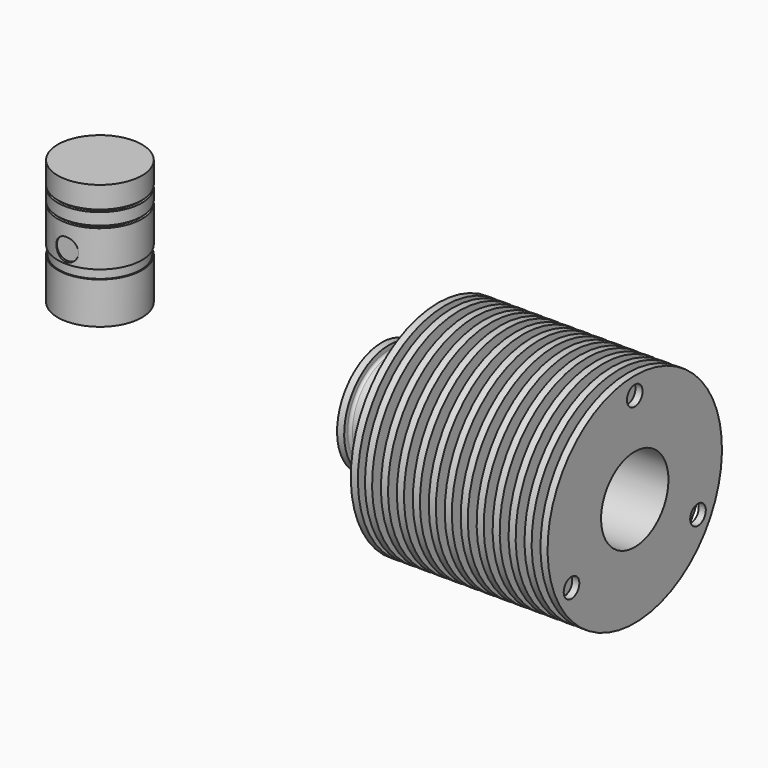
from build123d import *

# Parameters (mm, degrees)
F2_R      = 1.25
F3_DEPTH  = 5
F4_R      = 4.35
F5_DEPTH  = 4
F6_DEPTH  = 9.4
F7_R      = 1.25
F8_DEPTH  = 4.5
F12_D     = 2.2
F13_R     = 0.5
F14_DEPTH = 6.5
F16_R     = 0.5
F17_DEPTH = 6.5
F19_R     = 0.5
F20_DEPTH = 6.5


# Not quite as in the source:
# - a feature names something its author has since deleted; it is built from what else it names


with BuildPart() as f1:
    # F0 (on Front) → F1 (revolve)
    with BuildSketch(Plane.XZ):
        Polygon((-4.7528314651, -0.0212201326), (-0.0028314651, -0.0212201326), (-0.0028314651, 14.0787798674), (-4.7528314651, 14.0787798674), (-4.7528314651, 11.6291058475), (-4.6228314651, 11.4991058475), (-4.7528314651, 11.3691058475), (-4.7528314651, 10.0291058475), (-4.6228314651, 9.8991058475), (-4.7528314651, 9.7691058475), (-4.7528314651, 5.6787798674), (-4.6228314651, 5.6787798674), (-4.6228314651, 4.6787798674), (-4.7528314651, 4.6787798674), align=None)
    revolve(axis=Axis((-0.0028314651, 0, 3.8338128439), (0, 0, -1)))

    # F2 (on Front) → F3 (cut, symmetric)
    with BuildSketch(Plane.XZ):
        with Locations((0, 7.1287798674)):
            Circle(F2_R)
    extrude(amount=F3_DEPTH, both=True, mode=Mode.SUBTRACT)

    # F4 (on face) → F5 (cut)
    with BuildSketch(Plane(origin=(0, 0, -0.0212201326), x_dir=(1, 0, 0), z_dir=(0, 0, -1))):
        Circle(F4_R)
        with BuildLine():
            ThreePointArc((-2.8, 1), (-2.5071067812, 1.7071067812), (-1.8, 2))
            Line((-1.8, 2), (1.8, 2))
            ThreePointArc((1.8, 2), (2.5071067812, 1.7071067812), (2.8, 1))
            Line((2.8, 1), (2.8, -1))
            ThreePointArc((2.8, -1), (2.5071067812, -1.7071067812), (1.8, -2))
            Line((1.8, -2), (-1.8, -2))
            ThreePointArc((-1.8, -2), (-2.5071067812, -1.7071067812), (-2.8, -1))
            Line((-2.8, -1), (-2.8, 1))
        make_face(mode=Mode.SUBTRACT)
    extrude(amount=-F5_DEPTH, mode=Mode.SUBTRACT)

    # F6 (cut): a face of the model
    f6_faces = [f1.faces().sort_by_distance(p)[0] for p in [
        (0, 0, -0.0212201326),
    ]]
    extrude(f6_faces, amount=-F6_DEPTH, mode=Mode.SUBTRACT)


with BuildPart() as f8:
    # F7 (on Front) → F8 (new body, symmetric)
    with BuildSketch(Plane.XZ):
        with Locations((0, 7.1287798674)):
            Circle(F7_R)
    extrude(amount=F8_DEPTH, both=True)


with BuildPart() as f10:
    # F9 (on Front) → F10 (revolve)
    with BuildSketch(Plane.XZ):
        with BuildLine():
            Line((31.7983374715, 6.3), (31.7983374715, 4.75))
            Line((31.7983374715, 4.75), (60.3483374715, 4.75))
            Line((60.3483374715, 4.75), (60.3483374715, 12.3))
            Line((60.3483374715, 12.3), (59.5483374715, 12.3))
            Line((59.5483374715, 12.3), (59.5483374715, 6.75))
            Line((59.5483374715, 6.75), (58.5483374715, 6.75))
            Line((58.5483374715, 6.75), (58.5483374715, 12.3))
            Line((58.5483374715, 12.3), (57.7483374715, 12.3))
            Line((57.7483374715, 12.3), (57.7483374715, 6))
            Line((57.7483374715, 6), (56.7483374715, 6))
            Line((56.7483374715, 6), (56.7483374715, 12.3))
            Line((56.7483374715, 12.3), (55.9483374715, 12.3))
            Line((55.9483374715, 12.3), (55.9483374715, 6))
            Line((55.9483374715, 6), (54.9483374715, 6))
            Line((54.9483374715, 6), (54.9483374715, 12.3))
            Line((54.9483374715, 12.3), (54.1483374715, 12.3))
            Line((54.1483374715, 12.3), (54.1483374715, 6))
            Line((54.1483374715, 6), (53.1483374715, 6))
            Line((53.1483374715, 6), (53.1483374715, 12.3))
            Line((53.1483374715, 12.3), (52.3483374715, 12.3))
            Line((52.3483374715, 12.3), (52.3483374715, 6))
            Line((52.3483374715, 6), (51.3483374715, 6))
            Line((51.3483374715, 6), (51.3483374715, 12.3))
            Line((51.3483374715, 12.3), (50.5483374715, 12.3))
            Line((50.5483374715, 12.3), (50.5483374715, 6))
            Line((50.5483374715, 6), (49.5483374715, 6))
            Line((49.5483374715, 6), (49.5483374715, 12.3))
            Line((49.5483374715, 12.3), (48.7483374715, 12.3))
            Line((48.7483374715, 12.3), (48.7483374715, 6))
            Line((48.7483374715, 6), (47.7483374715, 6))
            Line((47.7483374715, 6), (47.7483374715, 12.3))
            Line((47.7483374715, 12.3), (46.9483374715, 12.3))
            Line((46.9483374715, 12.3), (46.9483374715, 6))
            Line((46.9483374715, 6), (45.9483374715, 6))
            Line((45.9483374715, 6), (45.9483374715, 12.3))
            Line((45.9483374715, 12.3), (45.1483374715, 12.3))
            Line((45.1483374715, 12.3), (45.1483374715, 6))
            Line((45.1483374715, 6), (44.1483374715, 6))
            Line((44.1483374715, 6), (44.1483374715, 12.3))
            Line((44.1483374715, 12.3), (43.3483374715, 12.3))
            Line((43.3483374715, 12.3), (43.3483374715, 6))
            Line((43.3483374715, 6), (42.3483374715, 6))
            Line((42.3483374715, 6), (42.3483374715, 12.3))
            Line((42.3483374715, 12.3), (41.5483374715, 12.3))
            Line((41.5483374715, 12.3), (41.5483374715, 6))
            Line((41.5483374715, 6), (40.5483374715, 6))
            Line((40.5483374715, 6), (40.5483374715, 12.3))
            Line((40.5483374715, 12.3), (40.2410296977, 12.3))
            Line((40.2410296977, 12.3), (39.7483374715, 12.3))
            Line((39.7483374715, 12.3), (39.7483374715, 6.75))
            Line((39.7483374715, 6.75), (38.9483374715, 6.75))
            Line((38.9483374715, 6.75), (38.9483374715, 12.3))
            Line((38.9483374715, 12.3), (38.1483374715, 12.3))
            Line((38.1483374715, 12.3), (38.1483374715, 5.8))
            ThreePointArc((38.1483374715, 5.8), (38.0604695058, 5.5878679656), (37.8483374715, 5.5))
            Line((37.8483374715, 5.5), (37.6483374715, 5.5))
            ThreePointArc((37.6483374715, 5.5), (37.4362054371, 5.5878679656), (37.3483374715, 5.8))
            Line((37.3483374715, 5.8), (37.3483374715, 6.3))
            Line((37.3483374715, 6.3), (36.5483374715, 6.3))
            Line((36.5483374715, 6.3), (36.5483374715, 5.8))
            ThreePointArc((36.5483374715, 5.8), (36.4604695058, 5.5878679656), (36.2483374715, 5.5))
            Line((36.2483374715, 5.5), (32.8983374715, 5.5))
            ThreePointArc((32.8983374715, 5.5), (32.6862054371, 5.5878679656), (32.5983374715, 5.8))
            Line((32.5983374715, 5.8), (32.5983374715, 6.3))
            Line((32.5983374715, 6.3), (31.7983374715, 6.3))
        make_face()
    revolve(axis=Axis((45.7656339545, 0, 0), (1, 0, 0)))

    # F12 (through all)
    with Locations(Plane.YZ.offset(60.3483374715)):
        with Locations((0, 10.3), (-8.920061659, -5.15), (8.920061659, -5.15)):
            Hole(F12_D / 2)

    # F13 (on Top) → F14 (cut, symmetric)
    with BuildSketch(Plane.XY):
        with Locations((35.3687927127, 0)):
            Circle(F13_R)
    extrude(amount=F14_DEPTH, both=True, mode=Mode.SUBTRACT)

    # F16 (on line) → F17 (cut, symmetric)
    with BuildSketch(Plane(origin=(0, 0, 0), x_dir=(-1, 0, 0), z_dir=(0, 0.8660254038, 0.5))):
        with Locations((-35.2983374715, 0)):
            Circle(F16_R)
    extrude(amount=F17_DEPTH, both=True, mode=Mode.SUBTRACT)

    # F19 (on line) → F20 (cut, symmetric)
    with BuildSketch(Plane(origin=(0, 0, 0), x_dir=(-1, 0, 0), z_dir=(0, 0.8571673007, -0.5150380749))):
        with Locations((-35.2983374715, 0)):
            Circle(F19_R)
    extrude(amount=F20_DEPTH, both=True, mode=Mode.SUBTRACT)


solid = Compound([f1.part, f8.part, f10.part])
